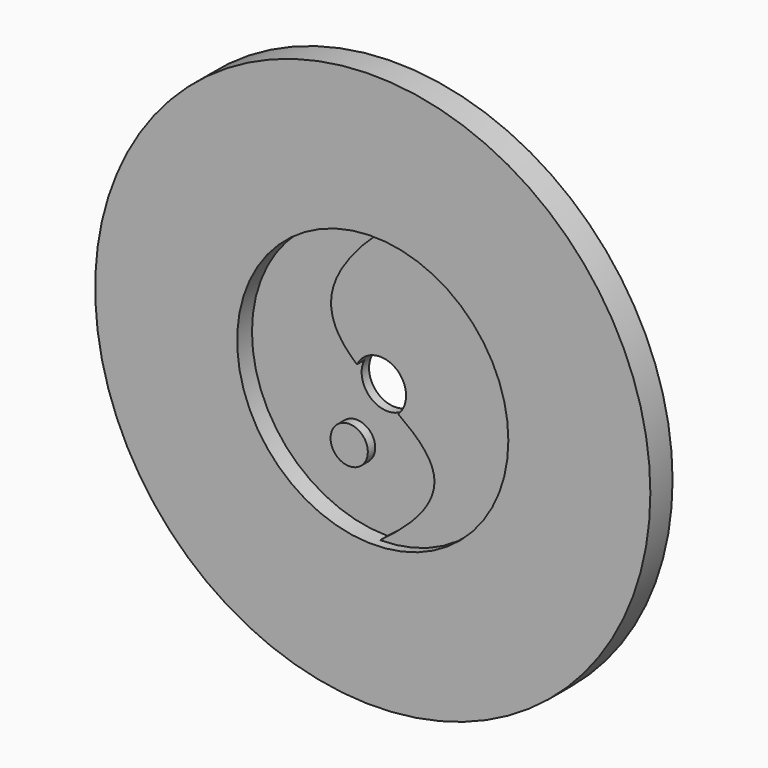
from build123d import *
from build123d import SkipClean  # not in build123d's __all__

# Parameters (mm, degrees)
F0_R     = 30
F0_R_2   = 2.8032876748
F1_DEPTH = 3
F2_R     = 14.6541534018
F2_R_2   = 2.8032876748
F3_DEPTH = 2
F5_DEPTH = 1
F6_R     = 2.0137101256
F7_DEPTH = 1


# Not quite as in the source:
# - after a boolean that leaves OpenCascade's solid faulty, fix() repairs it
# - the program builds the solid bodies; features that only make, move or delete a surface that nothing else refers to are left out


with BuildPart() as f1:
    # F0 (on Front) → F1 (new body)
    with BuildSketch(Plane.XZ):
        Circle(F0_R)
        Circle(F0_R_2, mode=Mode.SUBTRACT)
    extrude(amount=F1_DEPTH)

    # F2 (on face) → F3 (cut)
    with BuildSketch(Plane.XZ.offset(3)):
        Circle(F2_R)
        Circle(F2_R_2, mode=Mode.SUBTRACT)
    extrude(amount=-F3_DEPTH, mode=Mode.SUBTRACT)

    # F4 (on face) → F5 (join)
    with BuildSketch(Plane.XZ.offset(1)):
        with BuildLine():
            ThreePointArc((14.6541534018, 0), (10.362051243, 10.362051243), (0, 14.6541534018))
            add(Edge.make_bspline(
                [(0, 14.6541534018), (-7.4114441338, 7.865346928), (-5.8686273854, 4.1530740358), (-2.5122653336, 1.243762309)],
                knots=[0, 0, 0, 0, 11.5737184522, 11.5737184522, 11.5737184522, 11.5737184522], degree=3))
            ThreePointArc((-2.5122653336, 1.243762309), (0.6386780653, 2.7295626237), (2.8032876748, 0))
            ThreePointArc((2.8032876748, 0), (2.5797551305, -1.0969435967), (1.9448062102, -2.0189478924))
            add(Edge.make_bspline(
                [(1.9448062102, -2.0189478924), (6.0856305907, -4.9942852551), (8.8796933929, -8.1099972114), (0, -14.6541534018)],
                knots=[16.2199944228, 16.2199944228, 16.2199944228, 16.2199944228, 29.3083068036, 29.3083068036, 29.3083068036, 29.3083068036], degree=3))
            ThreePointArc((0, -14.6541534018), (10.362051243, -10.362051243), (14.6541534018, 0))
        make_face()
    with SkipClean():  # cleaning this boolean's faces spoils the solid; the shape is the same uncleaned
        extrude(amount=F5_DEPTH)

    # F6 (on face) → F7 (join)
    with BuildSketch(Plane.XZ.offset(1)):
        with Locations((-3.3478257246, -6.6966665909)):
            Circle(F6_R)
    extrude(amount=F7_DEPTH)

    add(f1.part.fix(), mode=Mode.REPLACE)


solid = f1.part
